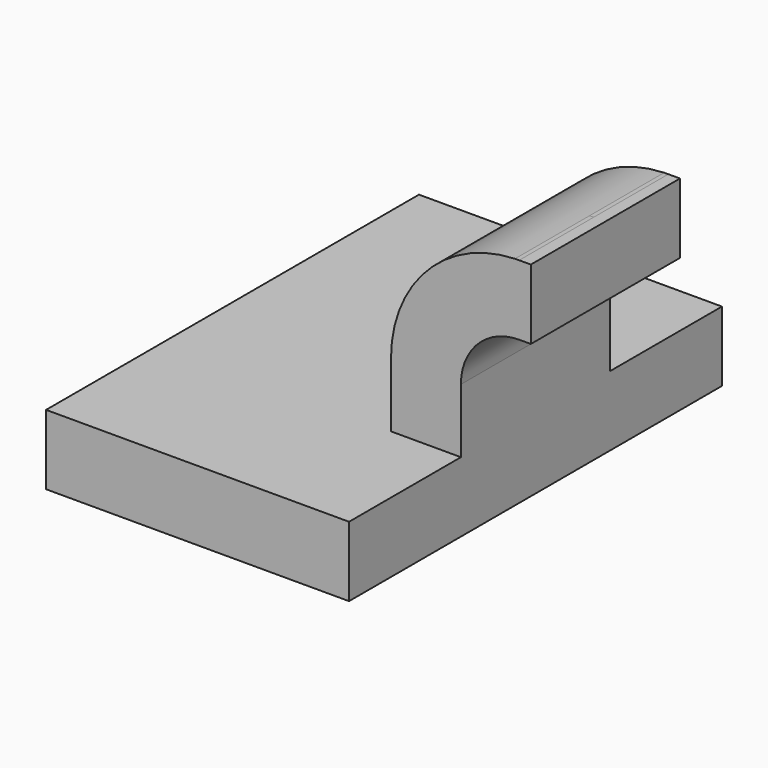
from build123d import *

# Parameters (mm, degrees)
F1_DEPTH = 63.5
F2_DEPTH = 25.4


# Not quite as in the source:
# - a feature of the source that left no trace in its solid (it failed there, or was rolled back) is left out


with BuildPart() as f1:
    # F0 (on Front) → F1 (new body, symmetric)
    with BuildSketch(Plane.XZ):
        Polygon((22.225, 12.7436925435), (-41.275, 12.7436925435), (-41.275, -6.3063074565), (41.275, -6.3063074565), (41.275, 12.7436925435), align=None)
    extrude(amount=F1_DEPTH, both=True)

    # F0 (on Front) → F2 (join, symmetric)
    with BuildSketch(Plane.XZ):
        with BuildLine():
            Line((22.225, 30.2188925435), (22.225, 12.7436925435))
            Line((22.225, 12.7436925435), (41.275, 12.7436925435))
            Line((41.275, 12.7436925435), (41.275, 30.2188925435))
            ThreePointArc((41.275, 30.2188925435), (45.9246798487, 41.4442126948), (57.15, 46.0938925435))
            Line((57.15, 46.0938925435), (60.325, 46.0938925435))
            Line((60.325, 46.0938925435), (60.325, 65.1438925435))
            Line((60.325, 65.1438925435), (57.15, 65.1438925435))
            add(Edge.make_bspline(
                [(57.15, 65.1438925435), (56.7668826582, 65.1373961276), (56.3837003417, 65.1310994591), (56.0004776373, 65.1249697126)],
                knots=[0, 0, 0, 0, 0.9177220122, 0.9177220122, 0.9177220122, 0.9177220122], degree=3))
            ThreePointArc((56.0004776373, 65.1249697126), (32.0511684185, 54.5047789437), (22.225, 30.2188925435))
        make_face()
    extrude(amount=F2_DEPTH, both=True)


solid = f1.part
